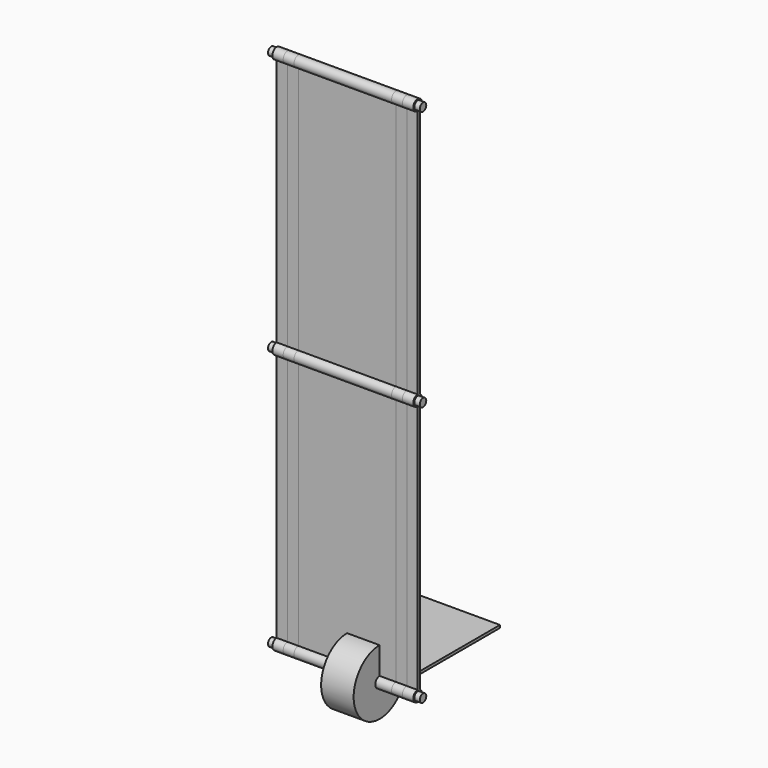
from build123d import *

# Parameters (mm, degrees)
F1_DEPTH = 114.3
F2_START = 114.3
F2_DEPTH = 25.4
F3_START = -114.3
F3_DEPTH = 25.4
F4_START = 139.7
F4_DEPTH = 25.4
F5_START = -139.7
F5_DEPTH = 25.4
F6_DEPTH = 177.8
F7_R     = 76.2
F8_DEPTH = 76.2


with BuildPart() as f1:
    # F0 (on Right) → F1 (new body, symmetric)
    with BuildSketch(Plane.YZ):
        with BuildLine():
            ThreePointArc((0, 622.3), (-12.7, 609.6), (0, 596.9))
            Line((0, 596.9), (0, 600.075))
            ThreePointArc((0, 600.075), (-9.525, 609.6), (0, 619.125))
            Line((0, 619.125), (0, 622.3))
        make_face()
        with BuildLine():
            ThreePointArc((10.998523, 6.35), (12.267258, 3.287002), (12.7, 0))
            Line((12.7, 0), (304.8, 0))
            Line((304.8, 0), (304.8, 6.35))
            Line((304.8, 6.35), (10.998523, 6.35))
        make_face()
        with BuildLine():
            Line((6.35, 602.500484), (6.35, 598.601477))
            ThreePointArc((6.35, 598.601477), (10.998523, 603.25), (12.7, 609.6))
            ThreePointArc((12.7, 609.6), (10.998523, 615.95), (6.35, 620.598523))
            Line((6.35, 620.598523), (6.35, 616.699516))
            ThreePointArc((6.35, 616.699516), (8.695096, 613.488565), (9.525, 609.6))
            ThreePointArc((9.525, 609.6), (8.695096, 605.711435), (6.35, 602.500484))
        make_face()
        with BuildLine():
            ThreePointArc((12.7, 1219.2), (-8.980256, 1228.180256), (0, 1206.5))
            Line((0, 1206.5), (0, 1209.675))
            ThreePointArc((0, 1209.675), (-6.735192, 1225.935192), (9.525, 1219.2))
            ThreePointArc((9.525, 1219.2), (8.695096, 1215.311435), (6.35, 1212.100484))
            Line((6.35, 1212.100484), (6.35, 1208.201477))
            ThreePointArc((6.35, 1208.201477), (10.998523, 1212.85), (12.7, 1219.2))
        make_face()
        with BuildLine():
            Line((0, 600.075), (0, 596.9))
            ThreePointArc((0, 596.9), (3.287002, 597.332742), (6.35, 598.601477))
            Line((6.35, 598.601477), (6.35, 602.500484))
            ThreePointArc((6.35, 602.500484), (3.39873, 600.702008), (0, 600.075))
        make_face()
        with BuildLine():
            Line((0, 596.9), (0, 12.7))
            ThreePointArc((0, 12.7), (3.287002, 12.267258), (6.35, 10.998523))
            Line((6.35, 10.998523), (6.35, 598.601477))
            ThreePointArc((6.35, 598.601477), (3.287002, 597.332742), (0, 596.9))
        make_face()
        with BuildLine():
            Line((0, 1209.675), (0, 1206.5))
            ThreePointArc((0, 1206.5), (3.287002, 1206.932742), (6.35, 1208.201477))
            Line((6.35, 1208.201477), (6.35, 1212.100484))
            ThreePointArc((6.35, 1212.100484), (3.39873, 1210.302008), (0, 1209.675))
        make_face()
        with BuildLine():
            Line((0, 1206.5), (0, 622.3))
            ThreePointArc((0, 622.3), (3.287002, 621.867258), (6.35, 620.598523))
            Line((6.35, 620.598523), (6.35, 1208.201477))
            ThreePointArc((6.35, 1208.201477), (3.287002, 1206.932742), (0, 1206.5))
        make_face()
        with BuildLine():
            ThreePointArc((6.35, 620.598523), (3.287002, 621.867258), (0, 622.3))
            Line((0, 622.3), (0, 619.125))
            ThreePointArc((0, 619.125), (3.39873, 618.497992), (6.35, 616.699516))
            Line((6.35, 616.699516), (6.35, 620.598523))
        make_face()
        with BuildLine():
            Line((0, 12.7), (0, 9.525))
            ThreePointArc((0, 9.525), (3.39873, 8.897992), (6.35, 7.099516))
            Line((6.35, 7.099516), (6.35, 10.998523))
            ThreePointArc((6.35, 10.998523), (3.287002, 12.267258), (0, 12.7))
        make_face()
        with BuildLine():
            Line((6.35, 10.998523), (6.35, 7.099516))
            ThreePointArc((6.35, 7.099516), (6.735192, 6.735192), (7.099516, 6.35))
            Line((7.099516, 6.35), (10.998523, 6.35))
            ThreePointArc((10.998523, 6.35), (8.980256, 8.980256), (6.35, 10.998523))
        make_face()
        with BuildLine():
            ThreePointArc((7.099516, 6.35), (8.897992, 3.39873), (9.525, 0))
            Line((9.525, 0), (12.7, 0))
            ThreePointArc((12.7, 0), (12.267258, 3.287002), (10.998523, 6.35))
            Line((10.998523, 6.35), (7.099516, 6.35))
        make_face()
        with BuildLine():
            ThreePointArc((9.525, 0), (-6.735192, -6.735192), (0, 9.525))
            Line((0, 9.525), (0, 12.7))
            ThreePointArc((0, 12.7), (-8.980256, -8.980256), (12.7, 0))
            Line((12.7, 0), (9.525, 0))
        make_face()
    extrude(amount=F1_DEPTH, both=True)


with BuildPart() as f2:
    # F0 (on Right) → F2 (new body)
    with BuildSketch(Plane.YZ.offset(F2_START)):
        with BuildLine():
            ThreePointArc((0, 622.3), (-12.7, 609.6), (0, 596.9))
            Line((0, 596.9), (0, 600.075))
            ThreePointArc((0, 600.075), (-9.525, 609.6), (0, 619.125))
            Line((0, 619.125), (0, 622.3))
        make_face()
        with BuildLine():
            Line((6.35, 10.998523), (6.35, 7.099516))
            ThreePointArc((6.35, 7.099516), (6.735192, 6.735192), (7.099516, 6.35))
            Line((7.099516, 6.35), (10.998523, 6.35))
            ThreePointArc((10.998523, 6.35), (8.980256, 8.980256), (6.35, 10.998523))
        make_face()
        with BuildLine():
            Line((6.35, 602.500484), (6.35, 598.601477))
            ThreePointArc((6.35, 598.601477), (10.998523, 603.25), (12.7, 609.6))
            ThreePointArc((12.7, 609.6), (10.998523, 615.95), (6.35, 620.598523))
            Line((6.35, 620.598523), (6.35, 616.699516))
            ThreePointArc((6.35, 616.699516), (8.695096, 613.488565), (9.525, 609.6))
            ThreePointArc((9.525, 609.6), (8.695096, 605.711435), (6.35, 602.500484))
        make_face()
        with BuildLine():
            ThreePointArc((12.7, 1219.2), (-8.980256, 1228.180256), (0, 1206.5))
            Line((0, 1206.5), (0, 1209.675))
            ThreePointArc((0, 1209.675), (-6.735192, 1225.935192), (9.525, 1219.2))
            ThreePointArc((9.525, 1219.2), (8.695096, 1215.311435), (6.35, 1212.100484))
            Line((6.35, 1212.100484), (6.35, 1208.201477))
            ThreePointArc((6.35, 1208.201477), (10.998523, 1212.85), (12.7, 1219.2))
        make_face()
        with BuildLine():
            ThreePointArc((6.35, 620.598523), (3.287002, 621.867258), (0, 622.3))
            Line((0, 622.3), (0, 619.125))
            ThreePointArc((0, 619.125), (3.39873, 618.497992), (6.35, 616.699516))
            Line((6.35, 616.699516), (6.35, 620.598523))
        make_face()
        with BuildLine():
            Line((0, 600.075), (0, 596.9))
            ThreePointArc((0, 596.9), (3.287002, 597.332742), (6.35, 598.601477))
            Line((6.35, 598.601477), (6.35, 602.500484))
            ThreePointArc((6.35, 602.500484), (3.39873, 600.702008), (0, 600.075))
        make_face()
        with BuildLine():
            ThreePointArc((9.525, 0), (-6.735192, -6.735192), (0, 9.525))
            Line((0, 9.525), (0, 12.7))
            ThreePointArc((0, 12.7), (-8.980256, -8.980256), (12.7, 0))
            Line((12.7, 0), (9.525, 0))
        make_face()
        with BuildLine():
            Line((0, 596.9), (0, 12.7))
            ThreePointArc((0, 12.7), (3.287002, 12.267258), (6.35, 10.998523))
            Line((6.35, 10.998523), (6.35, 598.601477))
            ThreePointArc((6.35, 598.601477), (3.287002, 597.332742), (0, 596.9))
        make_face()
        with BuildLine():
            Line((0, 1206.5), (0, 622.3))
            ThreePointArc((0, 622.3), (3.287002, 621.867258), (6.35, 620.598523))
            Line((6.35, 620.598523), (6.35, 1208.201477))
            ThreePointArc((6.35, 1208.201477), (3.287002, 1206.932742), (0, 1206.5))
        make_face()
        with BuildLine():
            Line((0, 12.7), (0, 9.525))
            ThreePointArc((0, 9.525), (3.39873, 8.897992), (6.35, 7.099516))
            Line((6.35, 7.099516), (6.35, 10.998523))
            ThreePointArc((6.35, 10.998523), (3.287002, 12.267258), (0, 12.7))
        make_face()
        with BuildLine():
            Line((0, 1209.675), (0, 1206.5))
            ThreePointArc((0, 1206.5), (3.287002, 1206.932742), (6.35, 1208.201477))
            Line((6.35, 1208.201477), (6.35, 1212.100484))
            ThreePointArc((6.35, 1212.100484), (3.39873, 1210.302008), (0, 1209.675))
        make_face()
        with BuildLine():
            ThreePointArc((7.099516, 6.35), (8.897992, 3.39873), (9.525, 0))
            Line((9.525, 0), (12.7, 0))
            ThreePointArc((12.7, 0), (12.267258, 3.287002), (10.998523, 6.35))
            Line((10.998523, 6.35), (7.099516, 6.35))
        make_face()
    extrude(amount=F2_DEPTH)


with BuildPart() as f3:
    # F0 (on Right) → F3 (new body)
    with BuildSketch(Plane.YZ.offset(F3_START)):
        with BuildLine():
            Line((6.35, 10.998523), (6.35, 7.099516))
            ThreePointArc((6.35, 7.099516), (6.735192, 6.735192), (7.099516, 6.35))
            Line((7.099516, 6.35), (10.998523, 6.35))
            ThreePointArc((10.998523, 6.35), (8.980256, 8.980256), (6.35, 10.998523))
        make_face()
        with BuildLine():
            Line((0, 12.7), (0, 9.525))
            ThreePointArc((0, 9.525), (3.39873, 8.897992), (6.35, 7.099516))
            Line((6.35, 7.099516), (6.35, 10.998523))
            ThreePointArc((6.35, 10.998523), (3.287002, 12.267258), (0, 12.7))
        make_face()
        with BuildLine():
            ThreePointArc((0, 622.3), (-12.7, 609.6), (0, 596.9))
            Line((0, 596.9), (0, 600.075))
            ThreePointArc((0, 600.075), (-9.525, 609.6), (0, 619.125))
            Line((0, 619.125), (0, 622.3))
        make_face()
        with BuildLine():
            ThreePointArc((12.7, 1219.2), (-8.980256, 1228.180256), (0, 1206.5))
            Line((0, 1206.5), (0, 1209.675))
            ThreePointArc((0, 1209.675), (-6.735192, 1225.935192), (9.525, 1219.2))
            ThreePointArc((9.525, 1219.2), (8.695096, 1215.311435), (6.35, 1212.100484))
            Line((6.35, 1212.100484), (6.35, 1208.201477))
            ThreePointArc((6.35, 1208.201477), (10.998523, 1212.85), (12.7, 1219.2))
        make_face()
        with BuildLine():
            Line((0, 596.9), (0, 12.7))
            ThreePointArc((0, 12.7), (3.287002, 12.267258), (6.35, 10.998523))
            Line((6.35, 10.998523), (6.35, 598.601477))
            ThreePointArc((6.35, 598.601477), (3.287002, 597.332742), (0, 596.9))
        make_face()
        with BuildLine():
            ThreePointArc((6.35, 620.598523), (3.287002, 621.867258), (0, 622.3))
            Line((0, 622.3), (0, 619.125))
            ThreePointArc((0, 619.125), (3.39873, 618.497992), (6.35, 616.699516))
            Line((6.35, 616.699516), (6.35, 620.598523))
        make_face()
        with BuildLine():
            Line((0, 1206.5), (0, 622.3))
            ThreePointArc((0, 622.3), (3.287002, 621.867258), (6.35, 620.598523))
            Line((6.35, 620.598523), (6.35, 1208.201477))
            ThreePointArc((6.35, 1208.201477), (3.287002, 1206.932742), (0, 1206.5))
        make_face()
        with BuildLine():
            Line((0, 1209.675), (0, 1206.5))
            ThreePointArc((0, 1206.5), (3.287002, 1206.932742), (6.35, 1208.201477))
            Line((6.35, 1208.201477), (6.35, 1212.100484))
            ThreePointArc((6.35, 1212.100484), (3.39873, 1210.302008), (0, 1209.675))
        make_face()
        with BuildLine():
            Line((0, 600.075), (0, 596.9))
            ThreePointArc((0, 596.9), (3.287002, 597.332742), (6.35, 598.601477))
            Line((6.35, 598.601477), (6.35, 602.500484))
            ThreePointArc((6.35, 602.500484), (3.39873, 600.702008), (0, 600.075))
        make_face()
        with BuildLine():
            Line((6.35, 602.500484), (6.35, 598.601477))
            ThreePointArc((6.35, 598.601477), (10.998523, 603.25), (12.7, 609.6))
            ThreePointArc((12.7, 609.6), (10.998523, 615.95), (6.35, 620.598523))
            Line((6.35, 620.598523), (6.35, 616.699516))
            ThreePointArc((6.35, 616.699516), (8.695096, 613.488565), (9.525, 609.6))
            ThreePointArc((9.525, 609.6), (8.695096, 605.711435), (6.35, 602.500484))
        make_face()
        with BuildLine():
            ThreePointArc((7.099516, 6.35), (8.897992, 3.39873), (9.525, 0))
            Line((9.525, 0), (12.7, 0))
            ThreePointArc((12.7, 0), (12.267258, 3.287002), (10.998523, 6.35))
            Line((10.998523, 6.35), (7.099516, 6.35))
        make_face()
        with BuildLine():
            ThreePointArc((9.525, 0), (-6.735192, -6.735192), (0, 9.525))
            Line((0, 9.525), (0, 12.7))
            ThreePointArc((0, 12.7), (-8.980256, -8.980256), (12.7, 0))
            Line((12.7, 0), (9.525, 0))
        make_face()
    extrude(amount=-F3_DEPTH)


with BuildPart() as f4:
    # F0 (on Right) → F4 (new body)
    with BuildSketch(Plane.YZ.offset(F4_START)):
        with BuildLine():
            Line((0, 1209.675), (0, 1206.5))
            ThreePointArc((0, 1206.5), (3.287002, 1206.932742), (6.35, 1208.201477))
            Line((6.35, 1208.201477), (6.35, 1212.100484))
            ThreePointArc((6.35, 1212.100484), (3.39873, 1210.302008), (0, 1209.675))
        make_face()
        with BuildLine():
            Line((0, 12.7), (0, 9.525))
            ThreePointArc((0, 9.525), (3.39873, 8.897992), (6.35, 7.099516))
            Line((6.35, 7.099516), (6.35, 10.998523))
            ThreePointArc((6.35, 10.998523), (3.287002, 12.267258), (0, 12.7))
        make_face()
        with BuildLine():
            Line((0, 600.075), (0, 596.9))
            ThreePointArc((0, 596.9), (3.287002, 597.332742), (6.35, 598.601477))
            Line((6.35, 598.601477), (6.35, 602.500484))
            ThreePointArc((6.35, 602.500484), (3.39873, 600.702008), (0, 600.075))
        make_face()
        with BuildLine():
            Line((6.35, 602.500484), (6.35, 598.601477))
            ThreePointArc((6.35, 598.601477), (10.998523, 603.25), (12.7, 609.6))
            ThreePointArc((12.7, 609.6), (10.998523, 615.95), (6.35, 620.598523))
            Line((6.35, 620.598523), (6.35, 616.699516))
            ThreePointArc((6.35, 616.699516), (8.695096, 613.488565), (9.525, 609.6))
            ThreePointArc((9.525, 609.6), (8.695096, 605.711435), (6.35, 602.500484))
        make_face()
        with BuildLine():
            ThreePointArc((6.35, 620.598523), (3.287002, 621.867258), (0, 622.3))
            Line((0, 622.3), (0, 619.125))
            ThreePointArc((0, 619.125), (3.39873, 618.497992), (6.35, 616.699516))
            Line((6.35, 616.699516), (6.35, 620.598523))
        make_face()
        with BuildLine():
            ThreePointArc((0, 622.3), (-12.7, 609.6), (0, 596.9))
            Line((0, 596.9), (0, 600.075))
            ThreePointArc((0, 600.075), (-9.525, 609.6), (0, 619.125))
            Line((0, 619.125), (0, 622.3))
        make_face()
        with BuildLine():
            Line((0, 596.9), (0, 12.7))
            ThreePointArc((0, 12.7), (3.287002, 12.267258), (6.35, 10.998523))
            Line((6.35, 10.998523), (6.35, 598.601477))
            ThreePointArc((6.35, 598.601477), (3.287002, 597.332742), (0, 596.9))
        make_face()
        with BuildLine():
            Line((0, 1206.5), (0, 622.3))
            ThreePointArc((0, 622.3), (3.287002, 621.867258), (6.35, 620.598523))
            Line((6.35, 620.598523), (6.35, 1208.201477))
            ThreePointArc((6.35, 1208.201477), (3.287002, 1206.932742), (0, 1206.5))
        make_face()
        with BuildLine():
            Line((6.35, 10.998523), (6.35, 7.099516))
            ThreePointArc((6.35, 7.099516), (6.735192, 6.735192), (7.099516, 6.35))
            Line((7.099516, 6.35), (10.998523, 6.35))
            ThreePointArc((10.998523, 6.35), (8.980256, 8.980256), (6.35, 10.998523))
        make_face()
        with BuildLine():
            ThreePointArc((12.7, 1219.2), (-8.980256, 1228.180256), (0, 1206.5))
            Line((0, 1206.5), (0, 1209.675))
            ThreePointArc((0, 1209.675), (-6.735192, 1225.935192), (9.525, 1219.2))
            ThreePointArc((9.525, 1219.2), (8.695096, 1215.311435), (6.35, 1212.100484))
            Line((6.35, 1212.100484), (6.35, 1208.201477))
            ThreePointArc((6.35, 1208.201477), (10.998523, 1212.85), (12.7, 1219.2))
        make_face()
        with BuildLine():
            ThreePointArc((7.099516, 6.35), (8.897992, 3.39873), (9.525, 0))
            Line((9.525, 0), (12.7, 0))
            ThreePointArc((12.7, 0), (12.267258, 3.287002), (10.998523, 6.35))
            Line((10.998523, 6.35), (7.099516, 6.35))
        make_face()
        with BuildLine():
            ThreePointArc((9.525, 0), (-6.735192, -6.735192), (0, 9.525))
            Line((0, 9.525), (0, 12.7))
            ThreePointArc((0, 12.7), (-8.980256, -8.980256), (12.7, 0))
            Line((12.7, 0), (9.525, 0))
        make_face()
    extrude(amount=F4_DEPTH)


with BuildPart() as f5:
    # F0 (on Right) → F5 (new body)
    with BuildSketch(Plane.YZ.offset(F5_START)):
        with BuildLine():
            Line((0, 12.7), (0, 9.525))
            ThreePointArc((0, 9.525), (3.39873, 8.897992), (6.35, 7.099516))
            Line((6.35, 7.099516), (6.35, 10.998523))
            ThreePointArc((6.35, 10.998523), (3.287002, 12.267258), (0, 12.7))
        make_face()
        with BuildLine():
            ThreePointArc((9.525, 0), (-6.735192, -6.735192), (0, 9.525))
            Line((0, 9.525), (0, 12.7))
            ThreePointArc((0, 12.7), (-8.980256, -8.980256), (12.7, 0))
            Line((12.7, 0), (9.525, 0))
        make_face()
        with BuildLine():
            Line((6.35, 10.998523), (6.35, 7.099516))
            ThreePointArc((6.35, 7.099516), (6.735192, 6.735192), (7.099516, 6.35))
            Line((7.099516, 6.35), (10.998523, 6.35))
            ThreePointArc((10.998523, 6.35), (8.980256, 8.980256), (6.35, 10.998523))
        make_face()
        with BuildLine():
            Line((0, 596.9), (0, 12.7))
            ThreePointArc((0, 12.7), (3.287002, 12.267258), (6.35, 10.998523))
            Line((6.35, 10.998523), (6.35, 598.601477))
            ThreePointArc((6.35, 598.601477), (3.287002, 597.332742), (0, 596.9))
        make_face()
        with BuildLine():
            ThreePointArc((6.35, 620.598523), (3.287002, 621.867258), (0, 622.3))
            Line((0, 622.3), (0, 619.125))
            ThreePointArc((0, 619.125), (3.39873, 618.497992), (6.35, 616.699516))
            Line((6.35, 616.699516), (6.35, 620.598523))
        make_face()
        with BuildLine():
            ThreePointArc((7.099516, 6.35), (8.897992, 3.39873), (9.525, 0))
            Line((9.525, 0), (12.7, 0))
            ThreePointArc((12.7, 0), (12.267258, 3.287002), (10.998523, 6.35))
            Line((10.998523, 6.35), (7.099516, 6.35))
        make_face()
        with BuildLine():
            Line((0, 600.075), (0, 596.9))
            ThreePointArc((0, 596.9), (3.287002, 597.332742), (6.35, 598.601477))
            Line((6.35, 598.601477), (6.35, 602.500484))
            ThreePointArc((6.35, 602.500484), (3.39873, 600.702008), (0, 600.075))
        make_face()
        with BuildLine():
            ThreePointArc((0, 622.3), (-12.7, 609.6), (0, 596.9))
            Line((0, 596.9), (0, 600.075))
            ThreePointArc((0, 600.075), (-9.525, 609.6), (0, 619.125))
            Line((0, 619.125), (0, 622.3))
        make_face()
        with BuildLine():
            Line((0, 1209.675), (0, 1206.5))
            ThreePointArc((0, 1206.5), (3.287002, 1206.932742), (6.35, 1208.201477))
            Line((6.35, 1208.201477), (6.35, 1212.100484))
            ThreePointArc((6.35, 1212.100484), (3.39873, 1210.302008), (0, 1209.675))
        make_face()
        with BuildLine():
            Line((0, 1206.5), (0, 622.3))
            ThreePointArc((0, 622.3), (3.287002, 621.867258), (6.35, 620.598523))
            Line((6.35, 620.598523), (6.35, 1208.201477))
            ThreePointArc((6.35, 1208.201477), (3.287002, 1206.932742), (0, 1206.5))
        make_face()
        with BuildLine():
            ThreePointArc((12.7, 1219.2), (-8.980256, 1228.180256), (0, 1206.5))
            Line((0, 1206.5), (0, 1209.675))
            ThreePointArc((0, 1209.675), (-6.735192, 1225.935192), (9.525, 1219.2))
            ThreePointArc((9.525, 1219.2), (8.695096, 1215.311435), (6.35, 1212.100484))
            Line((6.35, 1212.100484), (6.35, 1208.201477))
            ThreePointArc((6.35, 1208.201477), (10.998523, 1212.85), (12.7, 1219.2))
        make_face()
        with BuildLine():
            Line((6.35, 602.500484), (6.35, 598.601477))
            ThreePointArc((6.35, 598.601477), (10.998523, 603.25), (12.7, 609.6))
            ThreePointArc((12.7, 609.6), (10.998523, 615.95), (6.35, 620.598523))
            Line((6.35, 620.598523), (6.35, 616.699516))
            ThreePointArc((6.35, 616.699516), (8.695096, 613.488565), (9.525, 609.6))
            ThreePointArc((9.525, 609.6), (8.695096, 605.711435), (6.35, 602.500484))
        make_face()
    extrude(amount=-F5_DEPTH)


with BuildPart() as f6:
    # F0 (on Right) → F6 (new body, symmetric)
    with BuildSketch(Plane.YZ):
        with BuildLine():
            ThreePointArc((0, 619.125), (-9.525, 609.6), (0, 600.075))
            Line((0, 600.075), (0, 619.125))
        make_face()
        with BuildLine():
            Line((0, 619.125), (0, 600.075))
            ThreePointArc((0, 600.075), (3.39873, 600.702008), (6.35, 602.500484))
            Line((6.35, 602.500484), (6.35, 616.699516))
            ThreePointArc((6.35, 616.699516), (3.39873, 618.497992), (0, 619.125))
        make_face()
        with BuildLine():
            Line((6.35, 616.699516), (6.35, 602.500484))
            ThreePointArc((6.35, 602.500484), (8.695096, 605.711435), (9.525, 609.6))
            ThreePointArc((9.525, 609.6), (8.695096, 613.488565), (6.35, 616.699516))
        make_face()
    extrude(amount=F6_DEPTH, both=True)


with BuildPart() as f6b:
    # F0 (on Right) → F6, piece 2 (new body, symmetric)
    with BuildSketch(Plane.YZ):
        with BuildLine():
            Line((0, 1219.2), (0, 1209.675))
            ThreePointArc((0, 1209.675), (3.39873, 1210.302008), (6.35, 1212.100484))
            Line((6.35, 1212.100484), (6.35, 1219.2))
            Line((6.35, 1219.2), (0, 1219.2))
        make_face()
        with BuildLine():
            ThreePointArc((9.525, 1219.2), (-6.735192, 1225.935192), (0, 1209.675))
            Line((0, 1209.675), (0, 1219.2))
            Line((0, 1219.2), (6.35, 1219.2))
            Line((6.35, 1219.2), (6.35, 1212.100484))
            ThreePointArc((6.35, 1212.100484), (8.695096, 1215.311435), (9.525, 1219.2))
        make_face()
    extrude(amount=F6_DEPTH, both=True)


with BuildPart() as f6c:
    # F0 (on Right) → F6, piece 3 (new body, symmetric)
    with BuildSketch(Plane.YZ):
        with BuildLine():
            Line((9.525, 0), (0, 0))
            Line((0, 0), (0, 9.525))
            ThreePointArc((0, 9.525), (-6.735192, -6.735192), (9.525, 0))
        make_face()
        with BuildLine():
            Line((0, 9.525), (0, 0))
            Line((0, 0), (9.525, 0))
            ThreePointArc((9.525, 0), (8.897992, 3.39873), (7.099516, 6.35))
            Line((7.099516, 6.35), (6.35, 6.35))
            Line((6.35, 6.35), (6.35, 7.099516))
            ThreePointArc((6.35, 7.099516), (3.39873, 8.897992), (0, 9.525))
        make_face()
        with BuildLine():
            ThreePointArc((7.099516, 6.35), (6.735192, 6.735192), (6.35, 7.099516))
            Line((6.35, 7.099516), (6.35, 6.35))
            Line((6.35, 6.35), (7.099516, 6.35))
        make_face()
    extrude(amount=F6_DEPTH, both=True)


with BuildPart() as f8:
    # F7 (on Right) → F8 (new body)
    with BuildSketch(Plane.YZ):
        Circle(F7_R)
    extrude(amount=F8_DEPTH)


solid = Compound([f1.part, f2.part, f3.part, f4.part, f5.part, f6.part, f6b.part, f6c.part, f8.part])
